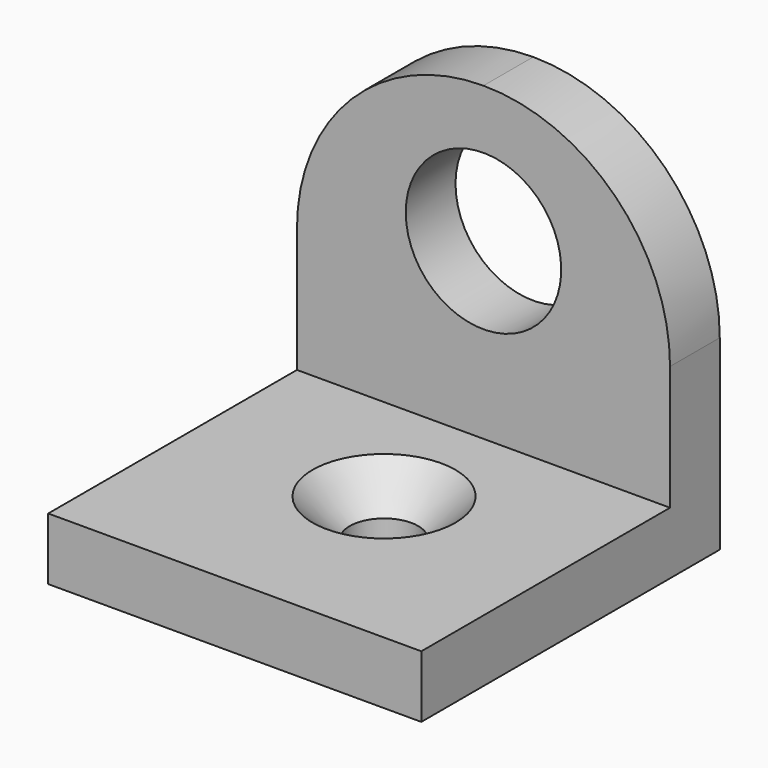
from build123d import *

# Parameters (mm, degrees)
F0_W     = 30
F0_H     = 30
F0_R     = 2.75
F1_DEPTH = 5
F2_W     = 30
F2_H     = 30
F3_DEPTH = 5
F4_R     = 6.25
F5_DEPTH = 6
F6_R     = 14.99999
F7_SIZE  = 3


# Not quite as in the source:
# - a fillet or chamfer is up to 0.001 mm smaller than in the source, because OpenCascade refuses the exact size


with BuildPart() as f1:
    # F0 (on Top) → F1 (new body)
    with BuildSketch(Plane.XY):
        with Locations((15, -1.7180653661)):
            Rectangle(F0_W, F0_H)
        with Locations((15, -1.7180653661)):
            Circle(F0_R, mode=Mode.SUBTRACT)
    extrude(amount=F1_DEPTH)

    # F2 (on face) → F3 (join)
    with BuildSketch(Plane(origin=(0, 13.2819346339, 0), x_dir=(-1, 0, 0), z_dir=(0, 1, 0))):
        with Locations((-15, 15)):
            Rectangle(F2_W, F2_H)
    extrude(amount=-F3_DEPTH)

    # F4 (on face) → F5 (cut)
    with BuildSketch(Plane(origin=(0, 13.2819346339, 0), x_dir=(-1, 0, 0), z_dir=(0, 1, 0))):
        with Locations((-15, 19)):
            Circle(F4_R)
    extrude(amount=-F5_DEPTH, mode=Mode.SUBTRACT)

    # F6 (radius 15 in the source; OpenCascade refuses exactly that, so slightly less here)
    f6_edges = [f1.edges().sort_by_distance(p)[0] for p in [
        (30, 10.781935, 30),
        (0, 10.781935, 30),
    ]]
    fillet(f6_edges, radius=F6_R)

    # F7
    f7_edges = [f1.edges().sort_by_distance(p)[0] for p in [
        (12.25, -1.718065, 5),
    ]]
    chamfer(f7_edges, length=F7_SIZE)


solid = f1.part
